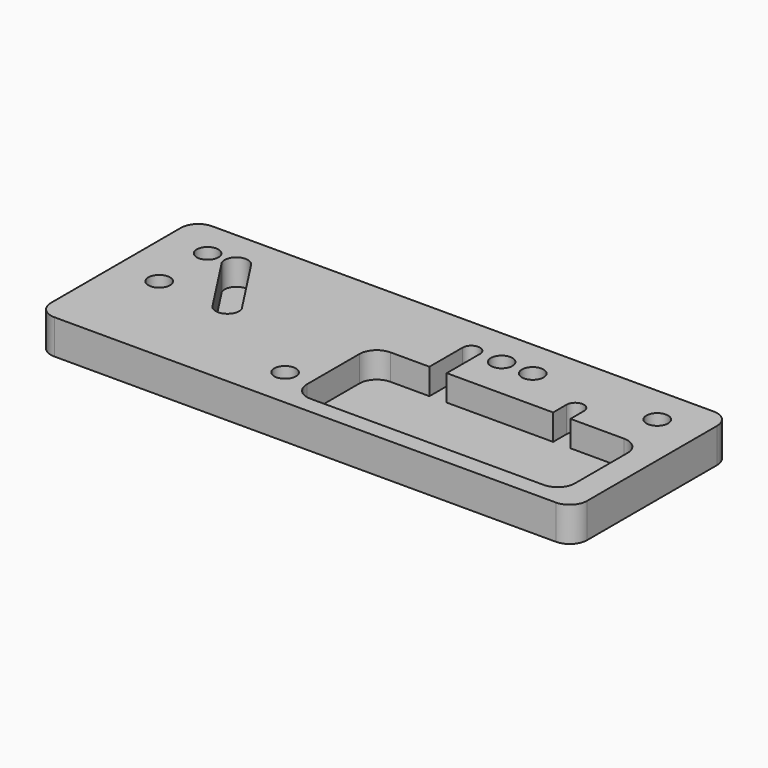
from build123d import *

# Parameters (mm, degrees)
F1_DEPTH = 25.4
F3_DEPTH = 19.05
F4_D     = 15.875
F4_DEPTH = 19.05
F4_TIP   = 4.7693311635


# Not quite as in the source:
# - a length typed as a fraction of an inch, garbled in the dataset ("3 / 203.2 mm" for 3/8 in), is restored


with BuildPart() as f1:
    # F0 (on Top) → F1 (new body)
    with BuildSketch(Plane.XY):
        with BuildLine():
            ThreePointArc((-196.85, -59.69), (-193.1302561211, -68.6702561211), (-184.15, -72.39))
            Line((-184.15, -72.39), (184.15, -72.39))
            ThreePointArc((184.15, -72.39), (193.1302561211, -68.6702561211), (196.85, -59.69))
            Line((196.85, -59.69), (196.85, 59.69))
            ThreePointArc((196.85, 59.69), (193.1302561211, 68.6702561211), (184.15, 72.39))
            Line((184.15, 72.39), (-184.15, 72.39))
            ThreePointArc((-184.15, 72.39), (-193.1302561211, 68.6702561211), (-196.85, 59.69))
            Line((-196.85, 59.69), (-196.85, -59.69))
        make_face()
    extrude(amount=-F1_DEPTH)

    # F2 (on Top) → F3 (cut)
    with BuildSketch(Plane.XY):
        with BuildLine():
            Line((22.1926261067, 13.97), (-6.35, 13.97))
            ThreePointArc((-6.35, 13.97), (-15.3302561211, 10.2502561211), (-19.05, 1.27))
            Line((-19.05, 1.27), (-19.05, -46.99))
            ThreePointArc((-19.05, -46.99), (-15.3302561211, -55.9702561211), (-6.35, -59.69))
            Line((-6.35, -59.69), (165.1, -59.69))
            ThreePointArc((165.1, -59.69), (174.0802561211, -55.9702561211), (177.8, -46.99))
            Line((177.8, -46.99), (177.8, 1.27))
            ThreePointArc((177.8, 1.27), (174.0802561211, 10.2502561211), (165.1, 13.97))
            Line((165.1, 13.97), (125.73, 13.97))
            Line((125.73, 13.97), (113.03, 13.97))
            Line((113.03, 13.97), (34.8926261067, 13.97))
            Line((34.8926261067, 13.97), (22.1926261067, 13.97))
        make_face()
        with BuildLine():
            Line((22.1926261067, 44.45), (22.1926261067, 13.97))
            Line((22.1926261067, 13.97), (34.8926261067, 13.97))
            Line((34.8926261067, 13.97), (34.8926261067, 44.45))
            ThreePointArc((34.8926261067, 44.45), (28.5426261067, 50.8), (22.1926261067, 44.45))
        make_face()
        with BuildLine():
            Line((113.03, 26.3348463923), (113.03, 13.97))
            Line((113.03, 13.97), (125.73, 13.97))
            Line((125.73, 13.97), (125.73, 26.3348463923))
            ThreePointArc((125.73, 26.3348463923), (119.38, 32.6848463923), (113.03, 26.3348463923))
        make_face()
        with BuildLine():
            ThreePointArc((-136.2642422318, 48.2357204892), (-147.6423993224, 51.8340887509), (-151.5906006098, 40.5725426972))
            Line((-151.5906006098, 40.5725426972), (-121.928781271, -5.026510451))
            ThreePointArc((-121.928781271, -5.026510451), (-110.8444944433, -8.0371380797), (-106.602422893, 2.636667341))
            Line((-106.602422893, 2.636667341), (-136.2642422318, 48.2357204892))
        make_face()
    extrude(amount=-F3_DEPTH, mode=Mode.SUBTRACT)

    # F4
    with Locations(Plane.XY):
        with Locations((-165.1, 44.45), (50.8, 44.45), (73.66, 44.45), (165.1, 44.45), (-165.1, 0), (-38.1, -43.18)):
            Hole(F4_D / 2, depth=F4_DEPTH)
            with Locations((0, 0, -(F4_DEPTH + F4_TIP / 2))):  # 118° drill point
                Cone(0, F4_D / 2, F4_TIP, mode=Mode.SUBTRACT)


solid = f1.part
